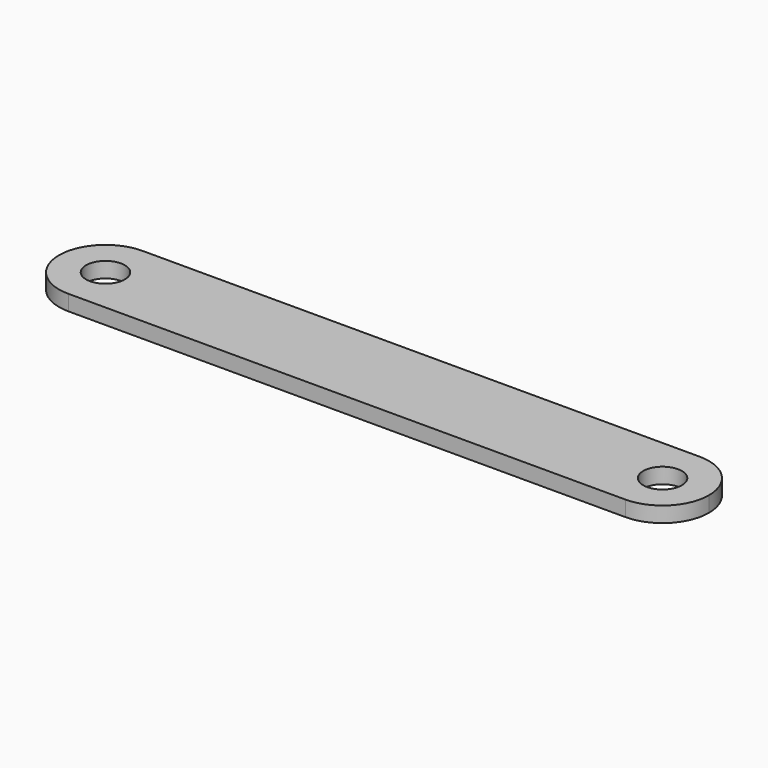
from build123d import *

# Parameters (mm, degrees)
F0_W     = 21
F0_H     = 3
F0_R     = 0.625
F1_DEPTH = 0.5
F2_R     = 1.49999


# Not quite as in the source:
# - a fillet or chamfer is up to 0.001 mm smaller than in the source, because OpenCascade refuses the exact size


with BuildPart() as f1:
    # F0 (on Top) → F1 (new body)
    with BuildSketch(Plane.XY):
        Rectangle(F0_W, F0_H)
        with Locations((-9, 0)):
            Circle(F0_R, mode=Mode.SUBTRACT)
        with Locations((9, 0)):
            Circle(F0_R, mode=Mode.SUBTRACT)
    extrude(amount=F1_DEPTH)

    # F2 (radius 1.5 in the source; OpenCascade refuses exactly that, so slightly less here)
    f2_edges = [f1.edges().sort_by_distance(p)[0] for p in [
        (-10.5, -1.5, 0.25),
        (-10.5, 1.5, 0.25),
        (10.5, -1.5, 0.25),
        (10.5, 1.5, 0.25),
    ]]
    fillet(f2_edges, radius=F2_R)


solid = f1.part
